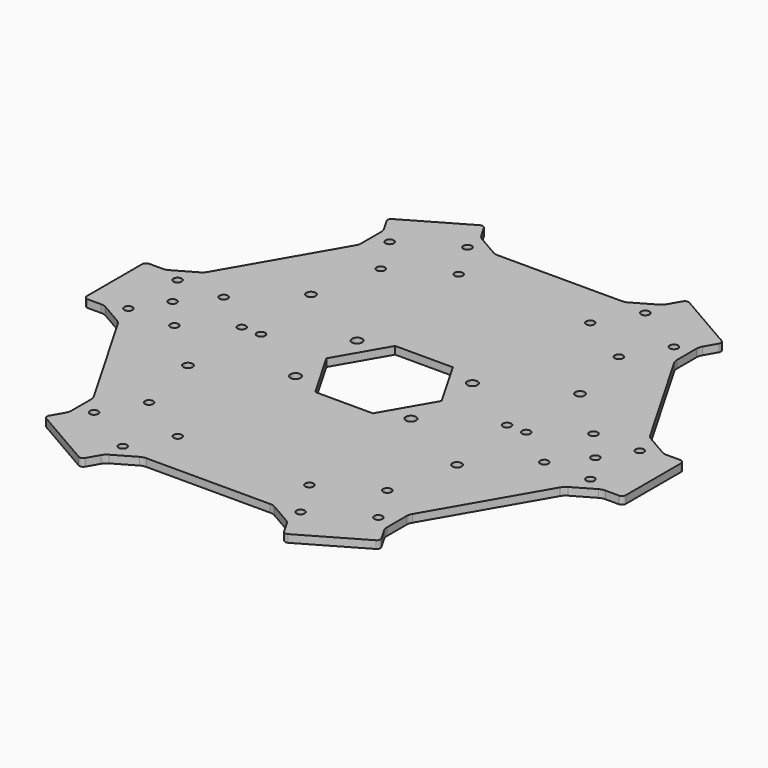
from build123d import *

# Parameters (mm, degrees)
F1_DEPTH        = 2
F2_R            = 3
F3_R            = 1
F5_D            = 2.15
F5_COPIES_COUNT = 6
F8_D            = 2.4
F10_D           = 2.65
F12_D           = 2.15
F12_DEPTH       = 4.05
F12_TIP         = 0.6459251655


# Not quite as in the source:
# - a pattern or mirror of a feature is missing from the dataset's text; its kind, count and spacing are read off the source's solid
# - a feature names something its author has since deleted; it is built from what else it names


with BuildPart() as f1:
    # F0 (on Top) → F1 (new body)
    with BuildSketch(Plane.XY):
        Polygon((16.9, 57.1576766498), (-16.9, 57.1576766498), (-23.7294919243, 61.1006856507), (-26.393684127, 65.7152019068), (-43.7141922027, 55.7152019068), (-41.05, 51.1006856507), (-41.05, 43.2146676488), (-57.95, 13.9430090009), (-64.7794919243, 10), (-70.1078763296, 10), (-70.1078763296, -10), (-64.7794919243, -10), (-57.95, -13.9430090009), (-41.05, -43.2146676488), (-41.05, -51.1006856507), (-43.7141922027, -55.7152019068), (-26.393684127, -65.7152019068), (-23.7294919243, -61.1006856507), (-16.9, -57.1576766498), (16.9, -57.1576766498), (23.7294919243, -61.1006856507), (26.393684127, -65.7152019068), (43.7141922027, -55.7152019068), (41.05, -51.1006856507), (41.05, -43.2146676488), (57.95, -13.9430090009), (64.7794919243, -10), (70.1078763296, -10), (70.1078763296, 10), (64.7794919243, 10), (57.95, 13.9430090009), (41.05, 43.2146676488), (41.05, 51.1006856507), (43.7141922027, 55.7152019068), (26.393684127, 65.7152019068), (23.7294919243, 61.1006856507), align=None)
        Polygon((-15, 0), (-7.5, 12.9903810568), (7.5, 12.9903810568), (15, 0), (7.5, -12.9903810568), (-7.5, -12.9903810568), align=None, mode=Mode.SUBTRACT)
    extrude(amount=F1_DEPTH)

    # F2
    f2_edges = [f1.edges().sort_by_distance(p)[0] for p in [
        (-16.9, -57.157677, 1),
        (-23.729492, -61.100686, 1),
        (16.9, -57.157677, 1),
        (23.729492, -61.100686, 1),
        (-41.05, -43.214668, 1),
        (-41.05, -51.100686, 1),
        (-57.95, -13.943009, 1),
        (-64.779492, -10, 1),
        (-64.779492, 10, 1),
        (-57.95, 13.943009, 1),
        (-41.05, 43.214668, 1),
        (-41.05, 51.100686, 1),
        (-16.9, 57.157677, 1),
        (-23.729492, 61.100686, 1),
        (16.9, 57.157677, 1),
        (23.729492, 61.100686, 1),
        (41.05, 43.214668, 1),
        (41.05, 51.100686, 1),
        (57.95, 13.943009, 1),
        (64.779492, 10, 1),
        (57.95, -13.943009, 1),
        (64.779492, -10, 1),
        (41.05, -51.100686, 1),
        (41.05, -43.214668, 1),
    ]]
    fillet(f2_edges, radius=F2_R)

    # F3
    f3_edges = [f1.edges().sort_by_distance(p)[0] for p in [
        (-26.393684, -65.715202, 1),
        (-43.714192, -55.715202, 1),
        (26.393684, -65.715202, 1),
        (43.714192, -55.715202, 1),
        (70.107876, -10, 1),
        (70.107876, 10, 1),
        (43.714192, 55.715202, 1),
        (26.393684, 65.715202, 1),
        (-26.393684, 65.715202, 1),
        (-43.714192, 55.715202, 1),
        (-70.107876, -10, 1),
        (-70.107876, 10, 1),
    ]]
    fillet(f3_edges, radius=F3_R)

    # F5 (through all)
    with Locations(Plane.XY.offset(2)):
        with Locations((60.1078763296, 8), (48.1078763296, 8), (48.1078763296, -8), (60.1078763296, -8)):
            f5 = Hole(F5_D / 2)

    # F5_copies: F5 ×6 about axis
    f5_copies_axis = Axis((0, 0, 0), (0, 0, 1))
    for i in range(1, F5_COPIES_COUNT):
        add(f5.rotate(f5_copies_axis, i * 360 / F5_COPIES_COUNT), mode=Mode.SUBTRACT)

    # F8 (through all)
    with Locations(Plane.XY.offset(2)):
        with Locations((-35, 20), (35, 20), (-35, -20), (35, -20)):
            Hole(F8_D / 2)

    # F10 (through all)
    with Locations(Plane.XY.offset(2)):
        with Locations((-15, 10), (15, 10), (15, -10), (-15, -10)):
            Hole(F10_D / 2)

    # F12
    with Locations(Plane.XY.offset(2)):
        with Locations((55, 0), (37, 0), (32, 0), (-32, 0), (-37, 0), (-55, 0)):
            Hole(F12_D / 2, depth=F12_DEPTH)
            with Locations((0, 0, -(F12_DEPTH + F12_TIP / 2))):  # 118° drill point
                Cone(0, F12_D / 2, F12_TIP, mode=Mode.SUBTRACT)


solid = f1.part
